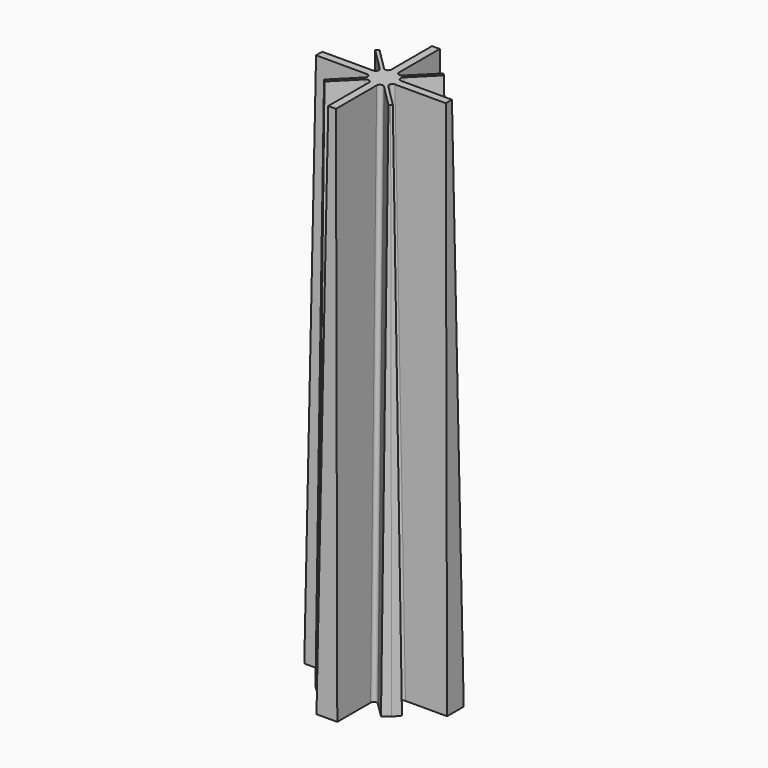
from build123d import *

# Parameters (mm, degrees)
F1_DEPTH               = 25
DRAFT_F1_DRAFTED_ANGLE = 0.7
F2_R                   = 0.15


# Not quite as in the source:
# - an extrude with a draft is written as a straight extrude whose walls are then drafted
# - a feature names something its author has since deleted; it is built from what else it names


with BuildPart() as f1:
    # F0 (on Top) → F1 (new body)
    with BuildSketch(Plane.XY):
        with BuildLine():
            Line((0.485925324, 3.3366640564), (0.25, 3.3366640564))
            Line((0.25, 3.3366640564), (0, 3.3366640564))
            Line((0, 3.3366640564), (-0.25, 3.3366640564))
            Line((-0.25, 3.3366640564), (-0.485925324, 3.3366640564))
            Line((-0.485925324, 3.3366640564), (-0.485925324, 2.4523206518))
            Line((-0.485925324, 2.4523206518), (-0.485925324, 1.0302226292))
            Line((-0.485925324, 1.0302226292), (-1.3355276656, 1.8798249708))
            Line((-1.3355276656, 1.8798249708), (-1.474543968, 2.0188412732))
            ThreePointArc((-1.474543968, 2.0188412732), (-1.6260087963, 1.8989721942), (-1.767766953, 1.767766953))
            ThreePointArc((-1.767766953, 1.767766953), (-1.8989721942, 1.6260087963), (-2.0188412732, 1.474543968))
            Line((-2.0188412732, 1.474543968), (-1.8798249708, 1.3355276656))
            Line((-1.8798249708, 1.3355276656), (-1.0302226292, 0.485925324))
            Line((-1.0302226292, 0.485925324), (-2.4523206518, 0.485925324))
            Line((-2.4523206518, 0.485925324), (-3.3366640564, 0.485925324))
            Line((-3.3366640564, 0.485925324), (-3.3366640564, 0.25))
            Line((-3.3366640564, 0.25), (-3.3366640564, 0))
            Line((-3.3366640564, 0), (-3.3366640564, -0.25))
            Line((-3.3366640564, -0.25), (-3.3366640564, -0.485925324))
            Line((-3.3366640564, -0.485925324), (-2.4523206518, -0.485925324))
            Line((-2.4523206518, -0.485925324), (-1.0302226292, -0.485925324))
            Line((-1.0302226292, -0.485925324), (-1.8798249708, -1.3355276656))
            Line((-1.8798249708, -1.3355276656), (-2.0188412732, -1.474543968))
            ThreePointArc((-2.0188412732, -1.474543968), (-1.8989721942, -1.6260087963), (-1.767766953, -1.767766953))
            ThreePointArc((-1.767766953, -1.767766953), (-1.6260087963, -1.8989721942), (-1.474543968, -2.0188412732))
            Line((-1.474543968, -2.0188412732), (-1.3355276656, -1.8798249708))
            Line((-1.3355276656, -1.8798249708), (-0.485925324, -1.0302226292))
            Line((-0.485925324, -1.0302226292), (-0.485925324, -2.4523206518))
            Line((-0.485925324, -2.4523206518), (-0.485925324, -3.3366640564))
            Line((-0.485925324, -3.3366640564), (-0.25, -3.3366640564))
            Line((-0.25, -3.3366640564), (0, -3.3366640564))
            Line((0, -3.3366640564), (0.25, -3.3366640564))
            Line((0.25, -3.3366640564), (0.485925324, -3.3366640564))
            Line((0.485925324, -3.3366640564), (0.485925324, -2.4523206518))
            Line((0.485925324, -2.4523206518), (0.485925324, -1.0302226292))
            Line((0.485925324, -1.0302226292), (1.3355276656, -1.8798249708))
            Line((1.3355276656, -1.8798249708), (1.474543968, -2.0188412732))
            ThreePointArc((1.474543968, -2.0188412732), (1.6260087963, -1.8989721942), (1.767766953, -1.767766953))
            ThreePointArc((1.767766953, -1.767766953), (1.8989721942, -1.6260087963), (2.0188412732, -1.474543968))
            Line((2.0188412732, -1.474543968), (1.8798249708, -1.3355276656))
            Line((1.8798249708, -1.3355276656), (1.0302226292, -0.485925324))
            Line((1.0302226292, -0.485925324), (2.4523206518, -0.485925324))
            Line((2.4523206518, -0.485925324), (3.3366640564, -0.485925324))
            Line((3.3366640564, -0.485925324), (3.3366640564, -0.25))
            Line((3.3366640564, -0.25), (3.3366640564, 0))
            Line((3.3366640564, 0), (3.3366640564, 0.25))
            Line((3.3366640564, 0.25), (3.3366640564, 0.485925324))
            Line((3.3366640564, 0.485925324), (2.4523206518, 0.485925324))
            Line((2.4523206518, 0.485925324), (1.0302226292, 0.485925324))
            Line((1.0302226292, 0.485925324), (1.8798249708, 1.3355276656))
            Line((1.8798249708, 1.3355276656), (2.0188412732, 1.474543968))
            ThreePointArc((2.0188412732, 1.474543968), (1.8989721942, 1.6260087963), (1.767766953, 1.767766953))
            ThreePointArc((1.767766953, 1.767766953), (1.6260087963, 1.8989721942), (1.474543968, 2.0188412732))
            Line((1.474543968, 2.0188412732), (1.3355276656, 1.8798249708))
            Line((1.3355276656, 1.8798249708), (0.485925324, 1.0302226292))
            Line((0.485925324, 1.0302226292), (0.485925324, 2.4523206518))
            Line((0.485925324, 2.4523206518), (0.485925324, 3.3366640564))
        make_face()
    extrude(amount=F1_DEPTH)

    # draft_F1_drafted
    draft_f1_drafted_walls = [f1.faces().sort_by_distance(p)[0] for p in [
        (0.980234646, 1.5245319512, 16.6666666667),
        (1.5245319512, 0.980234646, 16.6666666667),
        (2.1834433428, 0.485925324, 16.6666666667),
        (3.3366640564, 0, 16.6666666667),
        (2.1834433428, -0.485925324, 16.6666666667),
        (1.5245319512, -0.980234646, 16.6666666667),
        (1.767766953, -1.767766953, 16.6666666667),
        (0.980234646, -1.5245319512, 16.6666666667),
        (0.485925324, -2.1834433428, 16.6666666667),
        (0, -3.3366640564, 16.6666666667),
        (-0.485925324, -2.1834433428, 16.6666666667),
        (-0.980234646, -1.5245319512, 16.6666666667),
        (-1.767766953, -1.767766953, 16.6666666667),
        (-1.5245319512, -0.980234646, 16.6666666667),
        (-2.1834433428, -0.485925324, 16.6666666667),
        (-3.3366640564, 0, 16.6666666667),
        (-2.1834433428, 0.485925324, 16.6666666667),
        (-1.5245319512, 0.980234646, 16.6666666667),
        (-1.767766953, 1.767766953, 16.6666666667),
        (-0.980234646, 1.5245319512, 16.6666666667),
        (-0.485925324, 2.1834433428, 16.6666666667),
        (0, 3.3366640564, 16.6666666667),
        (0.485925324, 2.1834433428, 16.6666666667),
        (1.767766953, 1.767766953, 16.6666666667),
    ]]
    draft(draft_f1_drafted_walls, neutral_plane=Plane.XY, angle=DRAFT_F1_DRAFTED_ANGLE)

    # F2
    f2_edges = [f1.edges().sort_by_distance(p)[0] for p in [
        (0.333201, 0.661514, 12.5),
        (0.661514, 0.333201, 12.5),
        (0.661514, -0.333201, 12.5),
        (0.333201, -0.661514, 12.5),
        (-0.333201, -0.661514, 12.5),
        (-0.661514, -0.333201, 12.5),
        (-0.661514, 0.333201, 12.5),
        (-0.333201, 0.661514, 12.5),
    ]]
    fillet(f2_edges, radius=F2_R)


solid = f1.part
